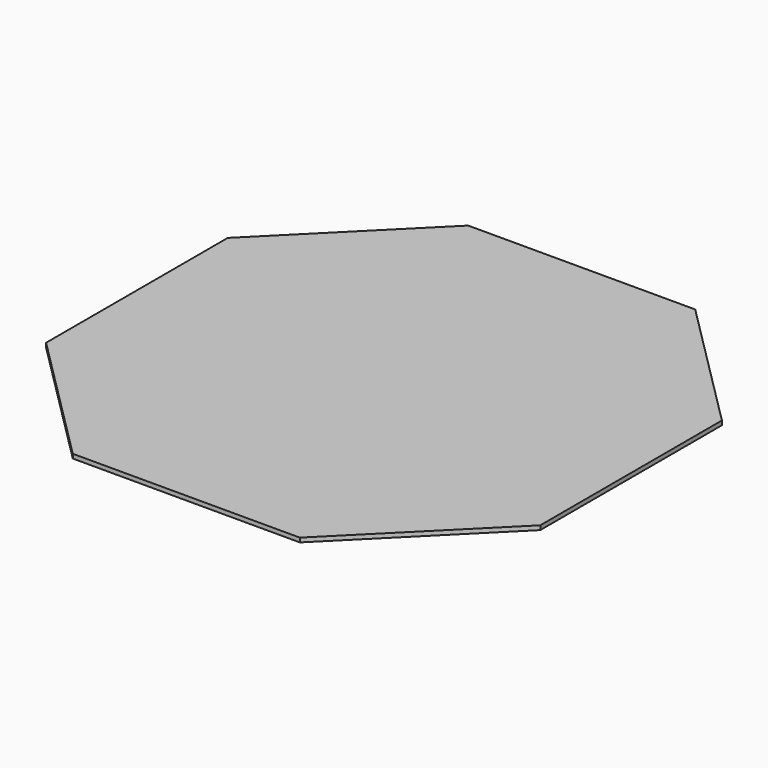
from build123d import *

# Parameters (mm, degrees)
F1_DEPTH = 3.175


# Not quite as in the source:
# - a length typed as a fraction of an inch, garbled in the dataset ("3 / 203.2 mm" for 3/8 in), is restored


with BuildPart() as f1:
    # F0 (on Top) → F1 (new body)
    with BuildSketch(Plane.XY):
        Polygon((-85, -185), (85, -185), (185, -85), (185, 85), (85, 185), (-85, 185), (-185, 85), (-185, -85), align=None)
    extrude(amount=F1_DEPTH)


solid = f1.part
